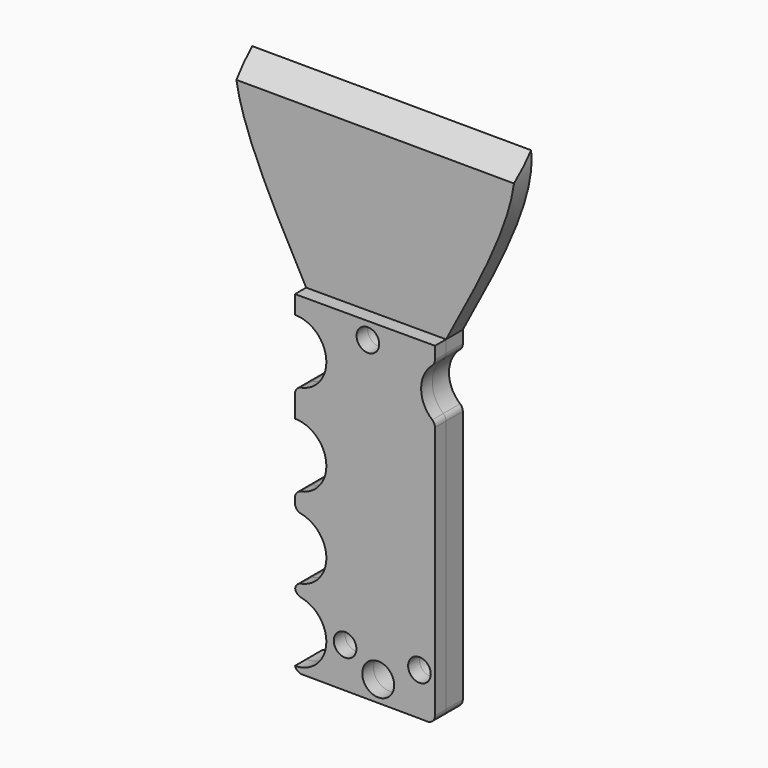
from build123d import *

# Parameters (mm, degrees)
F2_DEPTH    = 6
F3_T1_DEPTH = 115.827858657
F6_DEPTH    = 25
F7_T1_DEPTH = 15.7974131941
F7_T3_DEPTH = 16.290436999
F7_T5_DEPTH = 16.9242525679
F7_T7_DEPTH = 11.385777601
F9_DEPTH    = 4
F10_R       = 3.25
F10_R_2     = 4.5777520803
F11_DEPTH   = 25


# Not quite as in the source:
# - a fillet or chamfer that OpenCascade refuses, or shapes differently, is made with other operations: its cross-section is extruded or revolved along the edge and cut away or added


with BuildPart() as f2:
    # F1 (on face) → F2 (new body)
    with BuildSketch(Plane.XZ):
        with BuildLine():
            add(Edge.make_bspline(
                [(-20.9231331974, 46.4401495715), (-31.8316802492, 66.5727386597), (-42.740227301, 86.705327748), (-41.1091856658, 99.4347333908)],
                knots=[0, 0, 0, 0, 0.6149906941, 0.6149906941, 0.6149906941, 0.6149906941], degree=3))
            Line((-20.9231331974, 46.4401495715), (19.2433385447, 46.4401495715))
            add(Edge.make_bspline(
                [(19.2433385447, 46.4401495715), (30.0307332183, 66.6034940791), (40.8181278918, 86.7668385867), (38.7146398425, 99.160425365)],
                knots=[0, 0, 0, 0, 0.6129577408, 0.6129577408, 0.6129577408, 0.6129577408], degree=3))
            Line((38.7146398425, 99.160425365), (-41.1091856658, 99.4347333908))
        make_face()
        Polygon((19.2433385447, 46.4401495715), (-20.9231331974, 46.4401495715), (-20.9231331974, -48.9854468352), (19.2433385447, -49.2077428815), align=None)
    extrude(amount=F2_DEPTH)

    # F3: chamfer of 7 on 1 edges, made by hand

    # F3_s2 → F3_t1 (cut)
    with BuildSketch(Plane(origin=(56.3751046529, 0, -0.1937284209), x_dir=(0, 1, 0), z_dir=(-0.9999940956, 0, 0.0034363976))):
        Polygon((1, -99.2928787763), (-6, -92.2928787763), (-6, -99.2928787763), align=None)
    extrude(amount=F3_T1_DEPTH, mode=Mode.SUBTRACT)

    # F4 (on face) + F5 (on face) → F6 (cut)
    with BuildSketch(Plane.XZ.offset(6)):
        with BuildLine():
            ThreePointArc((-20.9231331974, 23.1888029575), (-14.5591721667, 25.8248419269), (-11.9231331974, 32.1888029575))
            ThreePointArc((-11.9231331974, 32.1888029575), (-14.5591721667, 38.5527639882), (-20.9231331974, 41.1888029575))
            Line((-20.9231331974, 41.1888029575), (-20.9231331974, 23.1888029575))
        make_face()
        with BuildLine():
            ThreePointArc((-11.9231331974, 5.9541198425), (-14.5591721667, 12.3180808732), (-20.9231331974, 14.9541198425))
            Line((-20.9231331974, 14.9541198425), (-20.9231331974, -3.0458801575))
            ThreePointArc((-20.9231331974, -3.0458801575), (-14.5591721667, -0.4098411882), (-11.9231331974, 5.9541198425))
        make_face()
        with BuildLine():
            ThreePointArc((-11.9231331974, -17.3358544707), (-14.5591721667, -10.9718934401), (-20.9231331974, -8.3358544707))
            Line((-20.9231331974, -8.3358544707), (-20.9231331974, -26.3358544707))
            ThreePointArc((-20.9231331974, -26.3358544707), (-14.5591721667, -23.6998155014), (-11.9231331974, -17.3358544707))
        make_face()
        with BuildLine():
            ThreePointArc((-11.9231331974, -38.484223187), (-14.5591721667, -32.1202621563), (-20.9231331974, -29.484223187))
            Line((-20.9231331974, -29.484223187), (-20.9231331974, -47.484223187))
            ThreePointArc((-20.9231331974, -47.484223187), (-14.5591721667, -44.8481842176), (-11.9231331974, -38.484223187))
        make_face()
    with BuildSketch(Plane.XZ.offset(6)):
        with BuildLine():
            Line((19.2433385447, 26.8704213686), (19.2433385447, 41.7904041223))
            ThreePointArc((19.2433385447, 41.7904041223), (15.2780707777, 34.3304127455), (19.2433385447, 26.8704213686))
        make_face()
    extrude(amount=-F6_DEPTH, mode=Mode.SUBTRACT)

    # F7: fillet of radius 2.1727922061 on 9 edges, made by hand

    # F7_s2 → F7_t1 (cut)
    with BuildSketch(Plane.XZ.offset(-4.898706597)):
        with BuildLine():
            ThreePointArc((-19.172887646, 23.3606298447), (-20.4294973343, 22.6082546705), (-20.9231331974, 21.2293203187))
            Line((-20.9231331974, 21.2293203187), (-20.9231331974, 23.1888029575))
            ThreePointArc((-20.9231331974, 23.1888029575), (-20.0438033433, 23.2318626871), (-19.172887646, 23.3606298447))
        make_face()
        with BuildLine():
            ThreePointArc((-19.172887646, -2.8740532703), (-20.4294973343, -3.6264284446), (-20.9231331974, -5.0053627963))
            Line((-20.9231331974, -5.0053627963), (-20.9231331974, -3.0458801575))
            ThreePointArc((-20.9231331974, -3.0458801575), (-20.0438033433, -3.0028204279), (-19.172887646, -2.8740532703))
        make_face()
        with BuildLine():
            ThreePointArc((-20.9231331974, -6.3763718319), (-20.4294973343, -7.7553061837), (-19.172887646, -8.5076813579))
            ThreePointArc((-19.172887646, -8.5076813579), (-20.0438033433, -8.3789142003), (-20.9231331974, -8.3358544707))
            Line((-20.9231331974, -8.3358544707), (-20.9231331974, -6.3763718319))
        make_face()
        with BuildLine():
            ThreePointArc((-19.172887646, -26.1640275835), (-20.4294973343, -26.9164027578), (-20.9231331974, -28.2953371095))
            Line((-20.9231331974, -28.2953371095), (-20.9231331974, -26.3358544707))
            ThreePointArc((-20.9231331974, -26.3358544707), (-20.0438033433, -26.2927947411), (-19.172887646, -26.1640275835))
        make_face()
        with BuildLine():
            ThreePointArc((-20.9231331974, -27.5247405482), (-20.4294973343, -28.9036748999), (-19.172887646, -29.6560500742))
            ThreePointArc((-19.172887646, -29.6560500742), (-20.0438033433, -29.5272829166), (-20.9231331974, -29.484223187))
            Line((-20.9231331974, -29.484223187), (-20.9231331974, -27.5247405482))
        make_face()
    extrude(amount=F7_T1_DEPTH, mode=Mode.SUBTRACT)

    # F7_s4 → F7_t3 (cut)
    with BuildSketch(Plane.XZ.offset(-5.1452184995)):
        with BuildLine():
            ThreePointArc((-20.9231331974, -47.484223187), (-20.1398278758, -48.5748592028), (-18.8650773156, -48.9968368743))
            Line((-18.8650773156, -48.9968368743), (-20.9231331974, -48.9854468352))
            Line((-20.9231331974, -48.9854468352), (-20.9231331974, -47.484223187))
        make_face()
    extrude(amount=F7_T3_DEPTH, mode=Mode.SUBTRACT)

    # F7_s6 → F7_t5 (cut)
    with BuildSketch(Plane.XZ.offset(-5.4621262839)):
        with BuildLine():
            ThreePointArc((17.0585214905, -49.1956512993), (18.6026851174, -48.5635340308), (19.2433385447, -47.0228923679))
            Line((19.2433385447, -47.0228923679), (19.2433385447, -49.2077428815))
            Line((19.2433385447, -49.2077428815), (17.0585214905, -49.1956512993))
        make_face()
    extrude(amount=F7_T5_DEPTH, mode=Mode.SUBTRACT)

    # F7_s8 → F7_t7 (cut)
    with BuildSketch(Plane.XZ.offset(-2.6928888005)):
        with BuildLine():
            ThreePointArc((19.2433385447, 42.8675596425), (19.0411479361, 41.9522698987), (18.4722060704, 41.2073259339))
            ThreePointArc((18.4722060704, 41.2073259339), (18.8499375305, 41.5092266762), (19.2433385447, 41.7904041223))
            Line((19.2433385447, 41.7904041223), (19.2433385447, 42.8675596425))
        make_face()
        with BuildLine():
            ThreePointArc((19.2433385447, 25.7932658484), (19.0411479361, 26.7085555922), (18.4722060704, 27.4534995571))
            ThreePointArc((18.4722060704, 27.4534995571), (18.8499375305, 27.1515988148), (19.2433385447, 26.8704213686))
            Line((19.2433385447, 26.8704213686), (19.2433385447, 25.7932658484))
        make_face()
    extrude(amount=F7_T7_DEPTH, mode=Mode.SUBTRACT)


with BuildPart() as f9:
    # F8 (on face) → F9 (new body)
    with BuildSketch(Plane.XZ.offset(6)):
        with BuildLine():
            Line((19.2433385447, 46.4401495715), (-20.9231331974, 46.4401495715))
            Line((-20.9231331974, 46.4401495715), (-20.9231331974, 41.1888029575))
            ThreePointArc((-20.9231331974, 41.1888029575), (-11.9661929269, 33.0681328116), (-19.172887646, 23.3606298447))
            ThreePointArc((-19.172887646, 23.3606298447), (-20.4294973343, 22.6082546704), (-20.9231331974, 21.2293203187))
            Line((-20.9231331974, 21.2293203187), (-20.9231331974, 14.9541198425))
            ThreePointArc((-20.9231331974, 14.9541198425), (-11.9661929269, 6.8334496966), (-19.172887646, -2.8740532703))
            ThreePointArc((-19.172887646, -2.8740532703), (-20.4294973343, -3.6264284446), (-20.9231331974, -5.0053627963))
            Line((-20.9231331974, -5.0053627963), (-20.9231331974, -6.3763718319))
            ThreePointArc((-20.9231331974, -6.3763718319), (-20.4294973343, -7.7553061836), (-19.172887646, -8.5076813579))
            ThreePointArc((-19.172887646, -8.5076813579), (-11.9231331974, -17.3358544707), (-19.172887646, -26.1640275836))
            ThreePointArc((-19.172887646, -26.1640275835), (-20.3000815705, -26.7724024071), (-20.888698119, -27.9100388289))
            ThreePointArc((-20.888698119, -27.9100388289), (-20.3000815705, -29.0476752506), (-19.172887646, -29.6560500742))
            ThreePointArc((-19.172887646, -29.6560500741), (-11.9661929269, -39.3635530411), (-20.9231331974, -47.484223187))
            ThreePointArc((-20.9231331974, -47.484223187), (-20.1398278758, -48.5748592028), (-18.8650773156, -48.9968368743))
            Line((-18.8650773156, -48.9968368743), (17.0585214905, -49.1956512993))
            ThreePointArc((17.0585214905, -49.1956512993), (18.6026851174, -48.5635340308), (19.2433385447, -47.0228923679))
            Line((19.2433385447, -47.0228923679), (19.2433385447, 25.7932658484))
            ThreePointArc((19.2433385447, 25.7932658484), (19.0411479361, 26.7085555922), (18.4722060704, 27.4534995571))
            ThreePointArc((18.4722060704, 27.4534995571), (15.2780707777, 34.3304127455), (18.4722060704, 41.2073259339))
            ThreePointArc((18.4722060704, 41.2073259339), (19.0411479361, 41.9522698987), (19.2433385447, 42.8675596425))
            Line((19.2433385447, 42.8675596425), (19.2433385447, 46.4401495715))
        make_face()
    extrude(amount=F9_DEPTH)


with BuildPart() as f11_tool:
    # F10 (on face) → F11 (new body)
    with BuildSketch(Plane.XZ.offset(10)):
        with Locations((0, 41.6379310191)):
            Circle(F10_R)
        with Locations((-6.5396036953, -37.4999977648)):
            Circle(F10_R)
        with Locations((2.9647059273, -43.124999851)):
            Circle(F10_R_2)
        with Locations((14.796603471, -36.9181036949)):
            Circle(F10_R)
    extrude(amount=-F11_DEPTH)


with BuildPart() as f2_1:
    add(f2.part)

    # F11: cut by f11_tool
    add(f11_tool.part, mode=Mode.SUBTRACT)


with BuildPart() as f9_1:
    add(f9.part)

    # F11: cut by f11_tool
    add(f11_tool.part, mode=Mode.SUBTRACT)


solid = Compound([f2_1.part, f9_1.part])
